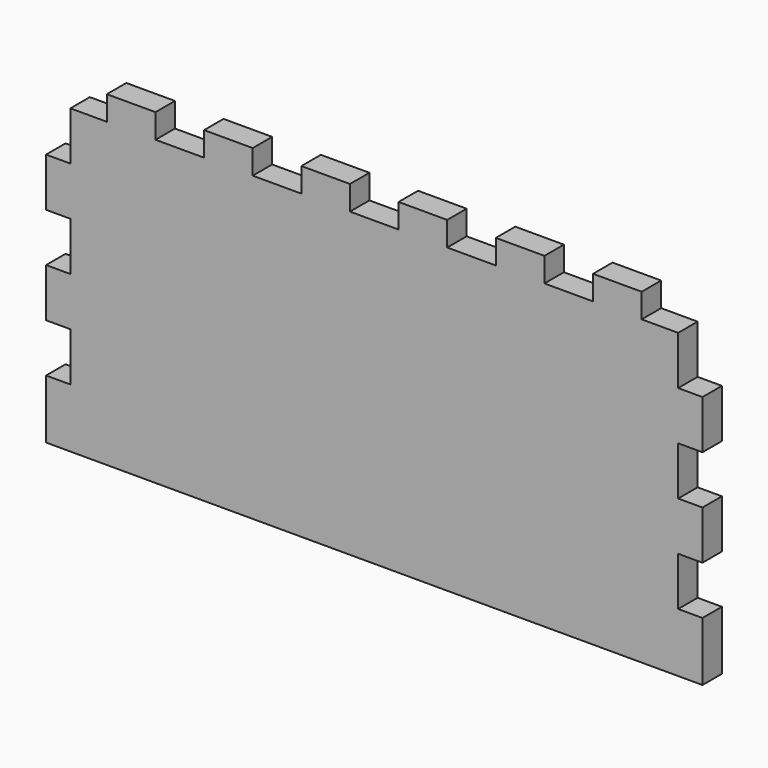
from build123d import *

# Parameters (mm, degrees)
F1_DEPTH = 10


# Not quite as in the source:
# - a feature names something its author has since deleted; it is built from what else it names


with BuildPart() as f1:
    # F0 (on Front) → F1 (new body)
    with BuildSketch(Plane.XZ):
        Polygon((135, -100), (135, -110), (115, -110), (115, -100), (95, -100), (95, -110), (75, -110), (75, -100), (55, -100), (55, -110), (35, -110), (35, -100), (15, -100), (15, -110), (0, -110), (0, -130), (-10, -130), (-10, -150), (0, -150), (0, -170), (-10, -170), (-10, -190), (0, -190), (0, -210), (-10, -210), (-10, -234.2857142857), (260, -234.2857142857), (260, -210), (250, -210), (250, -190), (260, -190), (260, -170), (250, -170), (250, -150), (260, -150), (260, -130), (250, -130), (250, -110), (235, -110), (235, -100), (215, -100), (215, -110), (195, -110), (195, -100), (175, -100), (175, -110), (155, -110), (155, -100), align=None)
    extrude(amount=-F1_DEPTH)


solid = f1.part
